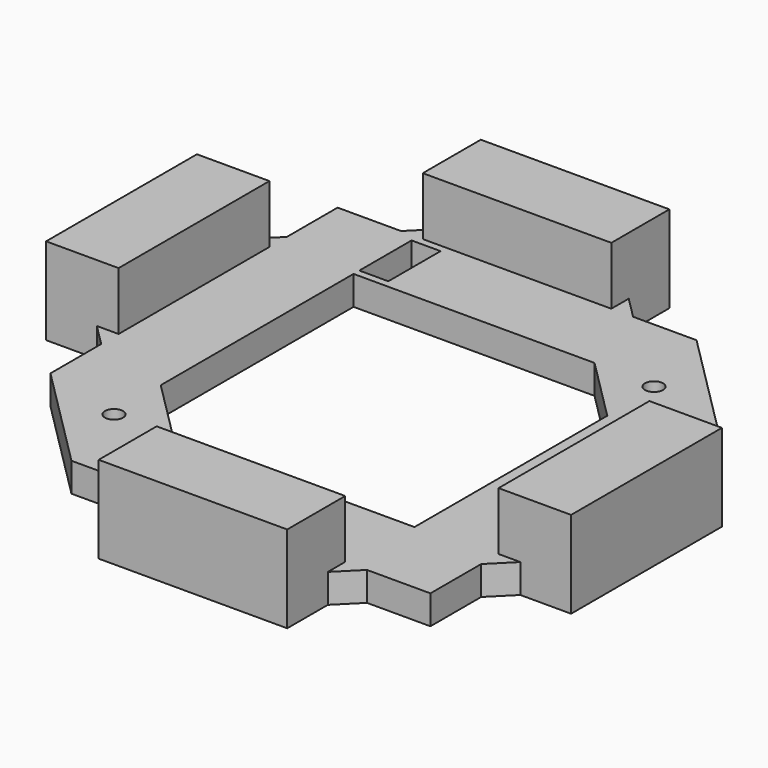
from build123d import *

# Parameters (mm, degrees)
F1_DEPTH = 4
F2_R     = 1.25
F3_DEPTH = 4.001
F4_W     = 4
F4_H     = 9
F5_DEPTH = 4.001
F6_W     = 10
F6_H     = 26
F6_W_2   = 26
F6_H_2   = 10
F7_DEPTH = 12
F8_SIZE  = 3


with BuildPart() as f1:
    # F0 (on Top) → F1 (new body)
    with BuildSketch(Plane.XY):
        Polygon((17.4974746831, 32), (-32, 32), (-32, -17.4974746831), (-17.4974746831, -32), (32, -32), (32, 17.4974746831), align=None)
        Polygon((-21, -12.2340187158), (-21, 21), (12.2340187158, 21), (21, 21), (21, 12.2340187158), (21, -21), (-12.2340187158, -21), (-21, -21), align=None, mode=Mode.SUBTRACT)
        Polygon((-12.2340187158, -21), (-21, -12.2340187158), (-21, -21), align=None)
        Polygon((21, 21), (12.2340187158, 21), (21, 12.2340187158), align=None)
    extrude(amount=F1_DEPTH)

    # F2 (on face) → F3 (cut, through all)
    with BuildSketch(Plane.XY.offset(4)):
        with Locations((-20.6828733497, -20.6828733497)):
            Circle(F2_R)
        with Locations((20.6828733497, 20.6828733497)):
            Circle(F2_R)
    extrude(amount=-F3_DEPTH, mode=Mode.SUBTRACT)

    # F4 (on face) → F5 (cut, through all)
    with BuildSketch(Plane.XY.offset(4)):
        with Locations((-19, 26.5)):
            Rectangle(F4_W, F4_H)
    extrude(amount=-F5_DEPTH, mode=Mode.SUBTRACT)

    # F6 (on face) → F7 (join)
    with BuildSketch(Plane(origin=(0, 0, 0), x_dir=(1, 0, 0), z_dir=(0, 0, -1))):
        with Locations((-37, -7.2512626585)):
            Rectangle(F6_W, F6_H)
        with Locations((7.2512626585, 37)):
            Rectangle(F6_W_2, F6_H_2)
        with Locations((37, 7.2512626585)):
            Rectangle(F6_W, F6_H)
        with Locations((-7.2512626585, -37)):
            Rectangle(F6_W_2, F6_H_2)
    extrude(amount=-F7_DEPTH)

    # F8
    f8_edges = [f1.edges().sort_by_distance(p)[0] for p in [
        (32, 5.748737, 2),
        (32, -20.251263, 2),
        (20.251263, -32, 2),
        (-5.748737, -32, 2),
        (-32, -5.748737, 2),
        (-32, 20.251263, 2),
        (-20.251263, 32, 2),
        (5.748737, 32, 2),
    ]]
    chamfer(f8_edges, length=F8_SIZE)


solid = f1.part
